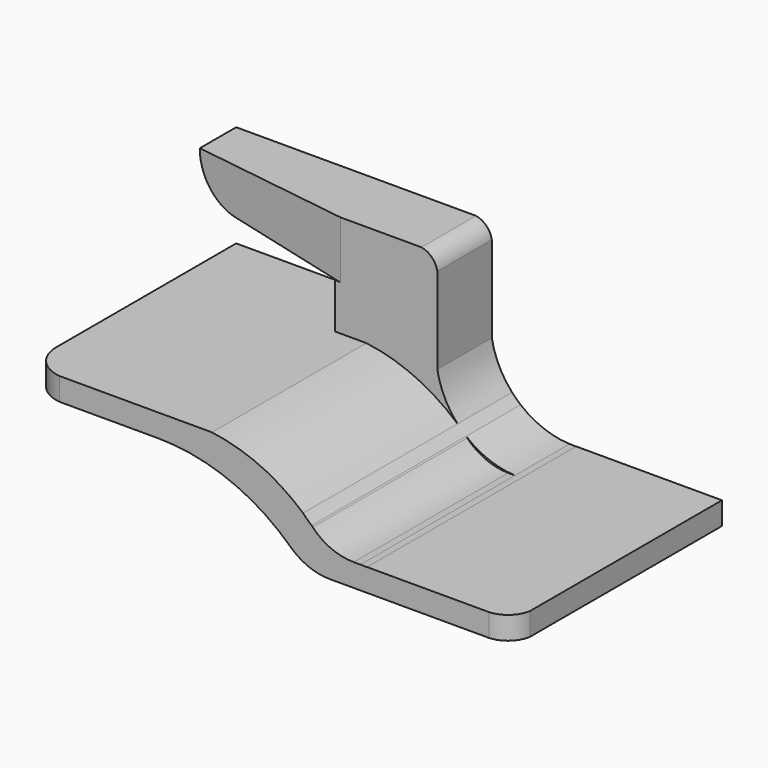
from build123d import *

# Parameters (mm, degrees)
F1_DEPTH  = 6
F2_DEPTH  = 23
F3_DEPTH  = 6
F4_R      = 5
F5_W      = 0.81186831
F5_H      = 2
F6_REACH  = 31.1431356237
F8_DEPTH  = 2
F10_DEPTH = 2
F11_R     = 5


with BuildPart() as f1:
    # F0 (on Front) → F1 (new body)
    with BuildSketch(Plane.XZ):
        with BuildLine():
            ThreePointArc((0, 22.7640915698), (-0.4760169509, 23.6848881741), (-1.3951592846, 24.1640915698))
            Line((-1.3951592846, 24.1640915698), (-22.5, 24.1640915698))
            ThreePointArc((-22.5, 24.1640915698), (-21.5061278282, 21.4707603394), (-18.9498743711, 20.1640915698))
            Line((-18.9498743711, 20.1640915698), (-9, 19.1640915698))
            Line((-9, 19.1640915698), (-9, 15.1640915698))
            Line((-9, 15.1640915698), (-6.2313233502, 15.1640915698))
            ThreePointArc((-6.2313233502, 15.1640915698), (-1.9506759829, 13.9418160027), (1.7829414728, 11.5173572715))
            ThreePointArc((1.7829414728, 11.5173572715), (0.6303147693, 13.2130414674), (0, 15.1640915698))
            Line((0, 15.1640915698), (0, 22.7640915698))
        make_face()
    extrude(amount=F1_DEPTH)

    # F0 (on Front) → F2 (join)
    with BuildSketch(Plane.XZ):
        with BuildLine():
            ThreePointArc((2.5376606134, 10.8007404291), (2.1473911285, 11.1454525194), (1.7829414728, 11.5173572715))
            ThreePointArc((1.7829414728, 11.5173572715), (-1.9506759829, 13.9418160027), (-6.2313233502, 15.1640915698))
            Line((-6.2313233502, 15.1640915698), (-9, 15.1640915698))
            Line((-9, 15.1640915698), (-22.5, 15.1640915698))
            Line((-22.5, 15.1640915698), (-22.5, 13.1640915698))
            Line((-22.5, 13.1640915698), (-11, 13.1640915698))
            ThreePointArc((-11, 13.1640915698), (-3.8410894684, 11.591731055), (2, 7.1640915698))
            Line((2, 7.1640915698), (20.2497988939, 7.1640915698))
            Line((20.2497988939, 7.1640915698), (20.2497988939, 9.1640915698))
            Line((20.2497988939, 9.1640915698), (7.4160159886, 9.1640915698))
            ThreePointArc((7.4160159886, 9.1640915698), (7.1261843392, 9.1582804924), (6.8363526899, 9.1640915698))
            Line((6.8363526899, 9.1640915698), (3.930054605, 9.1640915698))
            ThreePointArc((3.930054605, 9.1640915698), (3.2631933631, 10.0073736605), (2.5376606134, 10.8007404291))
        make_face()
    extrude(amount=F2_DEPTH)

    # F0 (on Front) → F3 (join)
    with BuildSketch(Plane.XZ):
        with BuildLine():
            ThreePointArc((6.8363526899, 9.1640915698), (4.5533954509, 9.6314834175), (2.5376606134, 10.8007404291))
            ThreePointArc((2.5376606134, 10.8007404291), (3.2631933631, 10.0073736605), (3.930054605, 9.1640915698))
            Line((3.930054605, 9.1640915698), (6.8363526899, 9.1640915698))
        make_face()
    extrude(amount=F3_DEPTH)

    # F4
    f4_edges = [f1.edges().sort_by_distance(p)[0] for p in [
        (3.930055, -14.5, 9.164092),
    ]]
    fillet(f4_edges, radius=F4_R)

    f6_end = Plane(origin=(-13.9749371855, -3, 19.6640915698), x_dir=(-0.9949874371, 0, 0.1), z_dir=(-0.1, 0, -0.9949874371))
    # F5 (on face) → F6 (cut, up to a plane its end follows)
    with BuildSketch(Plane.XY.offset(24.1640915698)):
        Polygon((-8.5, -6), (-22.5, -4), (-22.5, -6), align=None)
        with Locations((-22.905934155, -5)):
            Rectangle(F5_W, F5_H)
    f6_long = extrude(amount=-F6_REACH, mode=Mode.PRIVATE)
    add(split(f6_long, bisect_by=f6_end, keep=Keep.BOTTOM, mode=Mode.PRIVATE), mode=Mode.SUBTRACT)

    # F7 (on face) → F8 (cut, through all)
    with BuildSketch(Plane.XY.offset(15.1640915698)):
        with BuildLine():
            ThreePointArc((-19.6606274694, -23), (-21.6815784663, -21.9369160005), (-22.5, -19.8051147163))
            Line((-22.5, -19.8051147163), (-22.5, -23))
            Line((-22.5, -23), (-19.6606274694, -23))
        make_face()
    extrude(amount=-F8_DEPTH, mode=Mode.SUBTRACT)

    # F9 (on face) → F10 (cut, through all)
    with BuildSketch(Plane.XY.offset(9.1640915698)):
        with BuildLine():
            ThreePointArc((20.2497988939, -21.1107209325), (19.5387380379, -22.4279634054), (18.1554414653, -23))
            Line((18.1554414653, -23), (20.2497988939, -23))
            Line((20.2497988939, -23), (20.2497988939, -21.1107209325))
        make_face()
    extrude(amount=-F10_DEPTH, mode=Mode.SUBTRACT)

    # F11
    f11_edges = [f1.edges().sort_by_distance(p)[0] for p in [
        (2, -11.5, 7.164092),
    ]]
    fillet(f11_edges, radius=F11_R)


solid = f1.part
